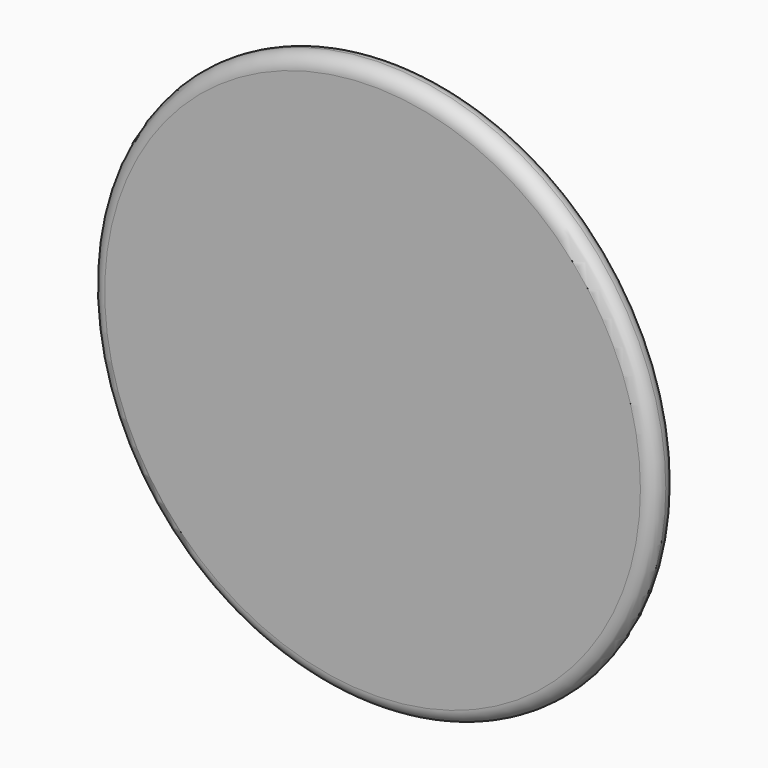
from build123d import *

# Parameters (mm, degrees)
F0_R     = 100
F1_DEPTH = 5
F2_R     = 4.99999


# Not quite as in the source:
# - a fillet or chamfer is up to 0.001 mm smaller than in the source, because OpenCascade refuses the exact size


with BuildPart() as f1:
    # F0 (on Front) → F1 (new body, symmetric)
    with BuildSketch(Plane.XZ):
        Circle(F0_R)
    extrude(amount=F1_DEPTH, both=True)

    # F2 (radius 5 in the source; OpenCascade refuses exactly that, so slightly less here)
    f2_edges = [f1.edges().sort_by_distance(p)[0] for p in [
        (-100, -5, 0),
        (-100, 5, 0),
    ]]
    fillet(f2_edges, radius=F2_R)


solid = f1.part
